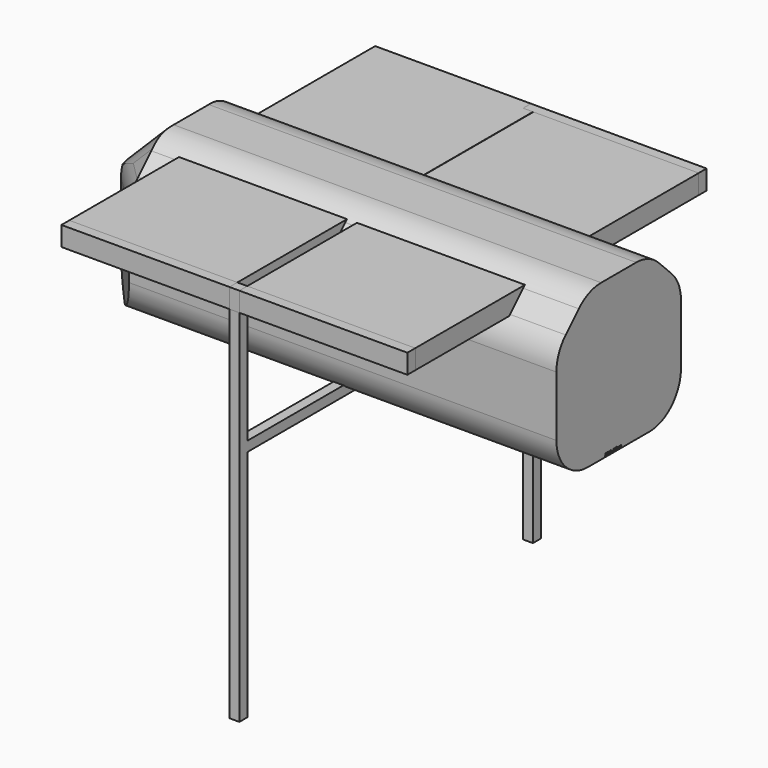
from build123d import *

# Parameters (mm, degrees)
F0_W          = 60
F0_H          = 20
F1_DEPTH      = 20
F3_DEPTH      = 15
F4_W          = 1.27
F4_H          = 1.2760577956
F5_DEPTH      = 15
F6_SIZE       = 5.08
F7_T1_DEPTH   = 65.4410244843
F7_T3_DEPTH   = 35.24
F7_T5_DEPTH   = 15.2572709248
F7_T7_DEPTH   = 15.2572709248
F7_T9_DEPTH   = 15.2572709248
F7_T14_DEPTH  = 37.62
F7_T19_DEPTH  = 37.62
F7_T24_DEPTH  = 50.32
F7_T31_DEPTH  = 50.32
F7_T37_DEPTH  = 50.32
F7_T43_DEPTH  = 54.13
F7_T49_DEPTH  = 54.13
F7_T55_DEPTH  = 54.13
F7_T62_DEPTH  = 41.43
F7_T67_DEPTH  = 41.43
F7_T72_DEPTH  = 49.0533849818
F7_T78_DEPTH  = 49.0533849818
F7_T84_DEPTH  = 49.0533849818
F7_T91_DEPTH  = 36.3533849818
F7_T96_DEPTH  = 36.3533849818
F7_T101_DEPTH = 55.4
F7_T107_DEPTH = 55.4
F7_T113_DEPTH = 55.4
F7_T120_DEPTH = 55.4
F7_T126_DEPTH = 55.4
F8_W          = 1.27
F8_H          = 1.2682774665
F9_DEPTH      = 15
F11_DEPTH     = 15
F12_W         = 21.5925588459
F12_H         = 1.2682774665
F13_DEPTH     = 2.5
F12_W_2       = 21.582525562
F14_DEPTH     = 2.5
F15_W         = 1.27
F15_H         = 1.2682774665
F16_DEPTH     = 2.5
F17_TEXT_SIZE = 0.4920971959
F18_DEPTH     = 0.0762
F20_W         = 0.5079289762
F20_H         = 6.7302512803
F21_DEPTH     = 0.3
F20_W_2       = 0.5036335206
F22_DEPTH     = 0.3
F20_W_3       = 0.5054401644
F23_DEPTH     = 0.3
F24_W         = 21.5925588459
F24_H         = 2.5
F25_DEPTH     = 25.4
F26_W         = 21.582525562
F26_H         = 2.5
F27_DEPTH     = 25.4
F29_DEPTH     = 2.5
F30_DEPTH     = 2.5
F31_W         = 1.2604115901
F31_H         = 2.5
F32_DEPTH     = 21.2852
F33_W         = 21.2420127096
F33_H         = 2.5
F34_DEPTH     = 25.4
F35_W         = 1.27
F35_H         = 1.2808652225
F36_DEPTH     = 30
F37_W         = 1.2666150182
F37_H         = 1.2703096864
F38_DEPTH     = 30


# Not quite as in the source:
# - a fillet or chamfer that OpenCascade refuses, or shapes differently, is made with other operations: its cross-section is extruded or revolved along the edge and cut away or added
# - two fillets or chamfers of one size are made in one step
# - Text() gives the source's letters only with a copy of the font that has no kerning and outlines rounded to 1/6400 em; it was checked with that copy


with BuildPart() as f1:
    # F0 (on Top) → F1 (new body)
    with BuildSketch(Plane.XY):
        with Locations((-42.5960034877, 2.3662830142)):
            Rectangle(F0_W, F0_H)
    extrude(amount=F1_DEPTH)

    # F2 (on face) → F3 (join)
    with BuildSketch(Plane(origin=(0, 12.3662830142, 0), x_dir=(-1, 0, 0), z_dir=(0, 1, 0))):
        Polygon((42.5873547792, 1.2760577956), (42.5960034877, 0), (43.862618506, 0), (43.862618506, 1.2760577956), align=None)
    extrude(amount=F3_DEPTH)

    # F4 (on face) → F5 (join)
    with BuildSketch(Plane.XZ.offset(7.6337169858)):
        with Locations((-41.9610034877, 0.6380288978)):
            Rectangle(F4_W, F4_H)
    extrude(amount=F5_DEPTH)

    # F6
    f6_edges = [f1.edges().sort_by_distance(p)[0] for p in [
        (-72.596003, 2.366283, 20),
        (-42.596003, -7.633717, 20),
        (-42.596003, 12.366283, 20),
        (-72.596003, 12.366283, 10),
        (-72.596003, -7.633717, 10),
    ]]
    chamfer(f6_edges, length=F6_SIZE)

    # F7: fillet of radius 5.08 on 13 edges, made by hand

    # F7_s2 → F7_t1 (cut)
    with BuildSketch(Plane.YZ.offset(-72.7765157298)):
        with BuildLine():
            ThreePointArc((5.1820781173, 20), (7.1261099537, 19.6133080252), (8.7741805657, 18.5121024484))
            Line((8.7741805657, 18.5121024484), (7.2862830142, 20))
            Line((7.2862830142, 20), (5.1820781173, 20))
        make_face()
        with BuildLine():
            ThreePointArc((12.3662830142, 12.8157951031), (11.9795910393, 14.7598269396), (10.8783854626, 16.4078975516))
            Line((10.8783854626, 16.4078975516), (12.3662830142, 14.92))
            Line((12.3662830142, 14.92), (12.3662830142, 12.8157951031))
        make_face()
        with BuildLine():
            ThreePointArc((-4.0416145374, 18.5121024484), (-2.3935439254, 19.6133080252), (-0.449512089, 20))
            Line((-0.449512089, 20), (-2.5537169858, 20))
            Line((-2.5537169858, 20), (-4.0416145374, 18.5121024484))
        make_face()
        with BuildLine():
            ThreePointArc((-7.6337169858, 12.8157951031), (-7.247025011, 14.7598269396), (-6.1458194343, 16.4078975516))
            Line((-6.1458194343, 16.4078975516), (-7.6337169858, 14.92))
            Line((-7.6337169858, 14.92), (-7.6337169858, 12.8157951031))
        make_face()
    extrude(amount=F7_T1_DEPTH, mode=Mode.SUBTRACT)

    # F7_s4 → F7_t3 (cut)
    with BuildSketch(Plane.XZ.offset(-19.9862830142)):
        with BuildLine():
            ThreePointArc((-67.5160034877, 0), (-71.1081059361, 1.4878975516), (-72.5960034877, 5.08))
            Line((-72.5960034877, 5.08), (-72.5960034877, 0))
            Line((-72.5960034877, 0), (-67.5160034877, 0))
        make_face()
    extrude(amount=F7_T3_DEPTH, mode=Mode.SUBTRACT)

    # F7_s6 → F7_t5 (cut)
    with BuildSketch(Plane(origin=(-27.0868833843, 27.0868833843, 0), x_dir=(0, 0, 1), z_dir=(-0.7071067812, 0.7071067812, 0))):
        with BuildLine():
            ThreePointArc((13.3053867944, -53.1388769511), (14.8441464628, -52.9002216696), (16.2383261619, -52.2066795822))
            Line((16.2383261619, -52.2066795822), (14.92, -53.1388769511))
            Line((14.92, -53.1388769511), (13.3053867944, -53.1388769511))
        make_face()
    extrude(amount=F7_T5_DEPTH, mode=Mode.SUBTRACT)

    # F7_s8 → F7_t7 (cut)
    with BuildSketch(Plane(origin=(-20.9037418772, 0, -20.9037418772), x_dir=(0, 1, 0), z_dir=(-0.7071067812, 0, -0.7071067812))):
        with BuildLine():
            ThreePointArc((-3.8720431477, -60.9509621596), (-2.4778634486, -61.644504247), (-0.9391037802, -61.8831595285))
            Line((-0.9391037802, -61.8831595285), (-2.5537169858, -61.8831595285))
            Line((-2.5537169858, -61.8831595285), (-3.8720431477, -60.9509621596))
        make_face()
        with BuildLine():
            ThreePointArc((5.6716698086, -61.8831595285), (7.2104294769, -61.644504247), (8.6046091761, -60.9509621596))
            Line((8.6046091761, -60.9509621596), (7.2862830142, -61.8831595285))
            Line((7.2862830142, -61.8831595285), (5.6716698086, -61.8831595285))
        make_face()
    extrude(amount=F7_T7_DEPTH, mode=Mode.SUBTRACT)

    # F7_s10 → F7_t9 (cut)
    with BuildSketch(Plane(origin=(-24.7206003701, -24.7206003701, 0), x_dir=(0, 0, 1), z_dir=(-0.7071067812, -0.7071067812, 0))):
        with BuildLine():
            ThreePointArc((13.3053867944, 56.4853064822), (14.8441464628, 56.2466512006), (16.2383261619, 55.5531091133))
            Line((16.2383261619, 55.5531091133), (14.92, 56.4853064822))
            Line((14.92, 56.4853064822), (13.3053867944, 56.4853064822))
        make_face()
    extrude(amount=F7_T9_DEPTH, mode=Mode.SUBTRACT)


with BuildPart() as f7_tool12:
    # F7_s13 → F7_t14 (new body)
    with BuildSketch(Plane.YZ.offset(-80.2160034877)):
        with BuildLine():
            ThreePointArc((-7.6337169858, 5.08), (-6.1458194343, 1.4878975516), (-2.5537169858, 0))
            Line((-2.5537169858, 0), (-7.6337169858, 0))
            Line((-7.6337169858, 0), (-7.6337169858, 5.08))
        make_face()
    extrude(amount=F7_T14_DEPTH)

    split(bisect_by=Plane.XY.offset(1.2760577956), keep=Keep.TOP)


with BuildPart() as f1_1:
    add(f1.part)

    # F7_t11: cut F7_tool12
    add(f7_tool12.part, mode=Mode.SUBTRACT)


with BuildPart() as f7_tool17:
    # F7_s18 → F7_t19 (new body)
    with BuildSketch(Plane.YZ.offset(-80.2160034877)):
        with BuildLine():
            ThreePointArc((-7.6337169858, 5.08), (-6.1458194343, 1.4878975516), (-2.5537169858, 0))
            Line((-2.5537169858, 0), (-7.6337169858, 0))
            Line((-7.6337169858, 0), (-7.6337169858, 5.08))
        make_face()
    extrude(amount=F7_T19_DEPTH)

    split(bisect_by=Plane.XY.offset(1.2760577956), keep=Keep.BOTTOM)


with BuildPart() as f1_2:
    add(f1_1.part)

    # F7_t16: cut F7_tool17
    add(f7_tool17.part, mode=Mode.SUBTRACT)


with BuildPart() as f7_tool22:
    # F7_s23 → F7_t24 (new body)
    with BuildSketch(Plane.YZ.offset(-80.2160034877)):
        with BuildLine():
            ThreePointArc((-7.6337169858, 5.08), (-6.1458194343, 1.4878975516), (-2.5537169858, 0))
            Line((-2.5537169858, 0), (-7.6337169858, 0))
            Line((-7.6337169858, 0), (-7.6337169858, 5.08))
        make_face()
    extrude(amount=F7_T24_DEPTH)

    split(bisect_by=Plane.YZ.offset(-42.5960034877), keep=Keep.TOP)

    split(bisect_by=Plane.XY.offset(1.2760577956), keep=Keep.TOP)

    split(bisect_by=Plane.YZ.offset(-41.3260034877), keep=Keep.BOTTOM)


with BuildPart() as f1_3:
    add(f1_2.part)

    # F7_t21: cut F7_tool22
    add(f7_tool22.part, mode=Mode.SUBTRACT)


with BuildPart() as f7_tool29:
    # F7_s30 → F7_t31 (new body)
    with BuildSketch(Plane.YZ.offset(-80.2160034877)):
        with BuildLine():
            ThreePointArc((-7.6337169858, 5.08), (-6.1458194343, 1.4878975516), (-2.5537169858, 0))
            Line((-2.5537169858, 0), (-7.6337169858, 0))
            Line((-7.6337169858, 0), (-7.6337169858, 5.08))
        make_face()
    extrude(amount=F7_T31_DEPTH)

    split(bisect_by=Plane.XY.offset(1.2760577956), keep=Keep.TOP)

    split(bisect_by=Plane.YZ.offset(-41.3260034877), keep=Keep.TOP)


with BuildPart() as f1_4:
    add(f1_3.part)

    # F7_t28: cut F7_tool29
    add(f7_tool29.part, mode=Mode.SUBTRACT)


with BuildPart() as f7_tool35:
    # F7_s36 → F7_t37 (new body)
    with BuildSketch(Plane.YZ.offset(-80.2160034877)):
        with BuildLine():
            ThreePointArc((-7.6337169858, 5.08), (-6.1458194343, 1.4878975516), (-2.5537169858, 0))
            Line((-2.5537169858, 0), (-7.6337169858, 0))
            Line((-7.6337169858, 0), (-7.6337169858, 5.08))
        make_face()
    extrude(amount=F7_T37_DEPTH)

    split(bisect_by=Plane.XY.offset(1.2760577956), keep=Keep.BOTTOM)

    split(bisect_by=Plane.YZ.offset(-41.3260034877), keep=Keep.TOP)


with BuildPart() as f1_5:
    add(f1_4.part)

    # F7_t34: cut F7_tool35
    add(f7_tool35.part, mode=Mode.SUBTRACT)


with BuildPart() as f7_tool41:
    # F7_s42 → F7_t43 (new body)
    with BuildSketch(Plane.YZ.offset(-54.0260034877)):
        with BuildLine():
            ThreePointArc((-7.6337169858, 5.08), (-6.1458194343, 1.4878975516), (-2.5537169858, 0))
            Line((-2.5537169858, 0), (-7.6337169858, 0))
            Line((-7.6337169858, 0), (-7.6337169858, 5.08))
        make_face()
    extrude(amount=F7_T43_DEPTH)

    split(bisect_by=Plane.YZ.offset(-42.5960034877), keep=Keep.BOTTOM)

    split(bisect_by=Plane.XY.offset(1.2760577956), keep=Keep.TOP)


with BuildPart() as f1_6:
    add(f1_5.part)

    # F7_t40: cut F7_tool41
    add(f7_tool41.part, mode=Mode.SUBTRACT)


with BuildPart() as f7_tool47:
    # F7_s48 → F7_t49 (new body)
    with BuildSketch(Plane.YZ.offset(-54.0260034877)):
        with BuildLine():
            ThreePointArc((-7.6337169858, 5.08), (-6.1458194343, 1.4878975516), (-2.5537169858, 0))
            Line((-2.5537169858, 0), (-7.6337169858, 0))
            Line((-7.6337169858, 0), (-7.6337169858, 5.08))
        make_face()
    extrude(amount=F7_T49_DEPTH)

    split(bisect_by=Plane.YZ.offset(-42.5960034877), keep=Keep.BOTTOM)

    split(bisect_by=Plane.XY.offset(1.2760577956), keep=Keep.BOTTOM)


with BuildPart() as f1_7:
    add(f1_6.part)

    # F7_t46: cut F7_tool47
    add(f7_tool47.part, mode=Mode.SUBTRACT)


with BuildPart() as f7_tool53:
    # F7_s54 → F7_t55 (new body)
    with BuildSketch(Plane.YZ.offset(-54.0260034877)):
        with BuildLine():
            ThreePointArc((-7.6337169858, 5.08), (-6.1458194343, 1.4878975516), (-2.5537169858, 0))
            Line((-2.5537169858, 0), (-7.6337169858, 0))
            Line((-7.6337169858, 0), (-7.6337169858, 5.08))
        make_face()
    extrude(amount=F7_T55_DEPTH)

    split(bisect_by=Plane.YZ.offset(-42.5960034877), keep=Keep.TOP)

    split(bisect_by=Plane.XY.offset(1.2760577956), keep=Keep.TOP)

    split(bisect_by=Plane.YZ.offset(-41.3260034877), keep=Keep.BOTTOM)


with BuildPart() as f1_8:
    add(f1_7.part)

    # F7_t52: cut F7_tool53
    add(f7_tool53.part, mode=Mode.SUBTRACT)


with BuildPart() as f7_tool60:
    # F7_s61 → F7_t62 (new body)
    with BuildSketch(Plane.YZ.offset(-41.3260034877)):
        with BuildLine():
            ThreePointArc((-7.6337169858, 5.08), (-6.1458194343, 1.4878975516), (-2.5537169858, 0))
            Line((-2.5537169858, 0), (-7.6337169858, 0))
            Line((-7.6337169858, 0), (-7.6337169858, 5.08))
        make_face()
    extrude(amount=F7_T62_DEPTH)

    split(bisect_by=Plane.XY.offset(1.2760577956), keep=Keep.TOP)


with BuildPart() as f1_9:
    add(f1_8.part)

    # F7_t59: cut F7_tool60
    add(f7_tool60.part, mode=Mode.SUBTRACT)


with BuildPart() as f7_tool65:
    # F7_s66 → F7_t67 (new body)
    with BuildSketch(Plane.YZ.offset(-41.3260034877)):
        with BuildLine():
            ThreePointArc((-7.6337169858, 5.08), (-6.1458194343, 1.4878975516), (-2.5537169858, 0))
            Line((-2.5537169858, 0), (-7.6337169858, 0))
            Line((-7.6337169858, 0), (-7.6337169858, 5.08))
        make_face()
    extrude(amount=F7_T67_DEPTH)

    split(bisect_by=Plane.XY.offset(1.2760577956), keep=Keep.BOTTOM)


with BuildPart() as f1_10:
    add(f1_9.part)

    # F7_t64: cut F7_tool65
    add(f7_tool65.part, mode=Mode.SUBTRACT)


with BuildPart() as f7_tool70:
    # F7_s71 → F7_t72 (new body)
    with BuildSketch(Plane.YZ.offset(-31.162618506)):
        with BuildLine():
            ThreePointArc((7.2862830142, 0), (10.8783854626, 1.4878975516), (12.3662830142, 5.08))
            Line((12.3662830142, 5.08), (12.3662830142, 0))
            Line((12.3662830142, 0), (7.2862830142, 0))
        make_face()
    extrude(amount=-F7_T72_DEPTH)

    split(bisect_by=Plane.XY.offset(1.2760577956), keep=Keep.BOTTOM)

    split(bisect_by=Plane(origin=(-42.5940468486, 0, 0.2886887214), x_dir=(0, 1, 0), z_dir=(0.9999770323, 0, -0.006777522)), keep=Keep.TOP)


with BuildPart() as f1_11:
    add(f1_10.part)

    # F7_t69: cut F7_tool70
    add(f7_tool70.part, mode=Mode.SUBTRACT)


with BuildPart() as f7_tool76:
    # F7_s77 → F7_t78 (new body)
    with BuildSketch(Plane.YZ.offset(-31.162618506)):
        with BuildLine():
            ThreePointArc((7.2862830142, 0), (10.8783854626, 1.4878975516), (12.3662830142, 5.08))
            Line((12.3662830142, 5.08), (12.3662830142, 0))
            Line((12.3662830142, 0), (7.2862830142, 0))
        make_face()
    extrude(amount=-F7_T78_DEPTH)

    split(bisect_by=Plane.XY.offset(1.2760577956), keep=Keep.TOP)

    split(bisect_by=Plane(origin=(-42.5940468486, 0, 0.2886887214), x_dir=(0, 1, 0), z_dir=(0.9999770323, 0, -0.006777522)), keep=Keep.TOP)


with BuildPart() as f1_12:
    add(f1_11.part)

    # F7_t75: cut F7_tool76
    add(f7_tool76.part, mode=Mode.SUBTRACT)


with BuildPart() as f7_tool82:
    # F7_s83 → F7_t84 (new body)
    with BuildSketch(Plane.YZ.offset(-31.162618506)):
        with BuildLine():
            ThreePointArc((7.2862830142, 0), (10.8783854626, 1.4878975516), (12.3662830142, 5.08))
            Line((12.3662830142, 5.08), (12.3662830142, 0))
            Line((12.3662830142, 0), (7.2862830142, 0))
        make_face()
    extrude(amount=-F7_T84_DEPTH)

    split(bisect_by=Plane.YZ.offset(-43.862618506), keep=Keep.TOP)

    split(bisect_by=Plane.XY.offset(1.2760577956), keep=Keep.TOP)

    split(bisect_by=Plane(origin=(-42.5940468486, 0, 0.2886887214), x_dir=(0, 1, 0), z_dir=(-0.9999770323, 0, 0.006777522)), keep=Keep.TOP)


with BuildPart() as f1_13:
    add(f1_12.part)

    # F7_t81: cut F7_tool82
    add(f7_tool82.part, mode=Mode.SUBTRACT)


with BuildPart() as f7_tool89:
    # F7_s90 → F7_t91 (new body)
    with BuildSketch(Plane.YZ.offset(-43.862618506)):
        with BuildLine():
            ThreePointArc((7.2862830142, 0), (10.8783854626, 1.4878975516), (12.3662830142, 5.08))
            Line((12.3662830142, 5.08), (12.3662830142, 0))
            Line((12.3662830142, 0), (7.2862830142, 0))
        make_face()
    extrude(amount=-F7_T91_DEPTH)

    split(bisect_by=Plane.XY.offset(1.2760577956), keep=Keep.BOTTOM)


with BuildPart() as f1_14:
    add(f1_13.part)

    # F7_t88: cut F7_tool89
    add(f7_tool89.part, mode=Mode.SUBTRACT)


with BuildPart() as f7_tool94:
    # F7_s95 → F7_t96 (new body)
    with BuildSketch(Plane.YZ.offset(-43.862618506)):
        with BuildLine():
            ThreePointArc((7.2862830142, 0), (10.8783854626, 1.4878975516), (12.3662830142, 5.08))
            Line((12.3662830142, 5.08), (12.3662830142, 0))
            Line((12.3662830142, 0), (7.2862830142, 0))
        make_face()
    extrude(amount=-F7_T96_DEPTH)

    split(bisect_by=Plane.XY.offset(1.2760577956), keep=Keep.TOP)


with BuildPart() as f1_15:
    add(f1_14.part)

    # F7_t93: cut F7_tool94
    add(f7_tool94.part, mode=Mode.SUBTRACT)


with BuildPart() as f7_tool99:
    # F7_s100 → F7_t101 (new body)
    with BuildSketch(Plane.YZ.offset(0.1039965123)):
        with BuildLine():
            ThreePointArc((7.2862830142, 0), (10.8783854626, 1.4878975516), (12.3662830142, 5.08))
            Line((12.3662830142, 5.08), (12.3662830142, 0))
            Line((12.3662830142, 0), (7.2862830142, 0))
        make_face()
    extrude(amount=-F7_T101_DEPTH)

    split(bisect_by=Plane.XY.offset(1.2760577956), keep=Keep.BOTTOM)

    split(bisect_by=Plane(origin=(-42.5940468486, 0, 0.2886887214), x_dir=(0, 1, 0), z_dir=(0.9999770323, 0, -0.006777522)), keep=Keep.TOP)


with BuildPart() as f1_16:
    add(f1_15.part)

    # F7_t98: cut F7_tool99
    add(f7_tool99.part, mode=Mode.SUBTRACT)


with BuildPart() as f7_tool105:
    # F7_s106 → F7_t107 (new body)
    with BuildSketch(Plane.YZ.offset(0.1039965123)):
        with BuildLine():
            ThreePointArc((7.2862830142, 0), (10.8783854626, 1.4878975516), (12.3662830142, 5.08))
            Line((12.3662830142, 5.08), (12.3662830142, 0))
            Line((12.3662830142, 0), (7.2862830142, 0))
        make_face()
    extrude(amount=-F7_T107_DEPTH)

    split(bisect_by=Plane.XY.offset(1.2760577956), keep=Keep.TOP)

    split(bisect_by=Plane(origin=(-42.5940468486, 0, 0.2886887214), x_dir=(0, 1, 0), z_dir=(0.9999770323, 0, -0.006777522)), keep=Keep.TOP)


with BuildPart() as f1_17:
    add(f1_16.part)

    # F7_t104: cut F7_tool105
    add(f7_tool105.part, mode=Mode.SUBTRACT)


with BuildPart() as f7_tool111:
    # F7_s112 → F7_t113 (new body)
    with BuildSketch(Plane.YZ.offset(0.1039965123)):
        with BuildLine():
            ThreePointArc((7.2862830142, 0), (10.8783854626, 1.4878975516), (12.3662830142, 5.08))
            Line((12.3662830142, 5.08), (12.3662830142, 0))
            Line((12.3662830142, 0), (7.2862830142, 0))
        make_face()
    extrude(amount=-F7_T113_DEPTH)

    split(bisect_by=Plane.YZ.offset(-43.862618506), keep=Keep.TOP)

    split(bisect_by=Plane.XY.offset(1.2760577956), keep=Keep.TOP)

    split(bisect_by=Plane(origin=(-42.5940468486, 0, 0.2886887214), x_dir=(0, 1, 0), z_dir=(-0.9999770323, 0, 0.006777522)), keep=Keep.TOP)


with BuildPart() as f1_18:
    add(f1_17.part)

    # F7_t110: cut F7_tool111
    add(f7_tool111.part, mode=Mode.SUBTRACT)


with BuildPart() as f7_tool118:
    # F7_s119 → F7_t120 (new body)
    with BuildSketch(Plane.YZ.offset(0.1039965123)):
        with BuildLine():
            ThreePointArc((7.2862830142, 0), (10.8783854626, 1.4878975516), (12.3662830142, 5.08))
            Line((12.3662830142, 5.08), (12.3662830142, 0))
            Line((12.3662830142, 0), (7.2862830142, 0))
        make_face()
    extrude(amount=-F7_T120_DEPTH)

    split(bisect_by=Plane.YZ.offset(-43.862618506), keep=Keep.BOTTOM)

    split(bisect_by=Plane.XY.offset(1.2760577956), keep=Keep.BOTTOM)


with BuildPart() as f1_19:
    add(f1_18.part)

    # F7_t117: cut F7_tool118
    add(f7_tool118.part, mode=Mode.SUBTRACT)


with BuildPart() as f7_tool124:
    # F7_s125 → F7_t126 (new body)
    with BuildSketch(Plane.YZ.offset(0.1039965123)):
        with BuildLine():
            ThreePointArc((7.2862830142, 0), (10.8783854626, 1.4878975516), (12.3662830142, 5.08))
            Line((12.3662830142, 5.08), (12.3662830142, 0))
            Line((12.3662830142, 0), (7.2862830142, 0))
        make_face()
    extrude(amount=-F7_T126_DEPTH)

    split(bisect_by=Plane.YZ.offset(-43.862618506), keep=Keep.BOTTOM)

    split(bisect_by=Plane.XY.offset(1.2760577956), keep=Keep.TOP)


with BuildPart() as f1_20:
    add(f1_19.part)

    # F7_t123: cut F7_tool124
    add(f7_tool124.part, mode=Mode.SUBTRACT)

    # F8 (on face) → F9 (join)
    with BuildSketch(Plane.XY.offset(1.2760577956)):
        with Locations((-41.9610034877, -21.9995782526)):
            Rectangle(F8_W, F8_H)
    extrude(amount=F9_DEPTH)

    # F10 (on face) → F11 (join)
    with BuildSketch(Plane.XY.offset(1.2760577956)):
        Polygon((-43.6347052455, 27.3662830142), (-43.862618506, 27.3662830142), (-43.862618506, 26.1058714241), (-42.5873547792, 26.1058714241), (-42.5873547792, 27.3662830142), align=None)
    extrude(amount=F11_DEPTH)

    # F17 (on face) → F18 (join)
    with BuildSketch(Plane.YZ.offset(-12.5960034877)):
        with Locations((0.1588490704, 0.0860145883)):
            Text('Allah Akbar', F17_TEXT_SIZE, font='Open Sans', text_align=(TextAlign.LEFT, TextAlign.BOTTOM))
    extrude(amount=F18_DEPTH)

    # F20 (on face) → F21 (join)
    with BuildSketch(Plane(origin=(-72.5960034877, 0, 0), x_dir=(0, -1, 0), z_dir=(-1, 0, 0))):
        with Locations((-5.4177053205, 9.9402611543)):
            Rectangle(F20_W, F20_H)
    extrude(amount=F21_DEPTH)

    # F20 (on face) → F22 (join)
    with BuildSketch(Plane(origin=(-72.5960034877, 0, 0), x_dir=(0, -1, 0), z_dir=(-1, 0, 0))):
        with Locations((-2.0122149144, 9.9402611543)):
            Rectangle(F20_W_2, F20_H)
    extrude(amount=F22_DEPTH)

    # F20 (on face) → F23 (join)
    with BuildSketch(Plane(origin=(-72.5960034877, 0, 0), x_dir=(0, -1, 0), z_dir=(-1, 0, 0))):
        with Locations((1.1918238625, 9.9402611543)):
            Rectangle(F20_W_3, F20_H)
    extrude(amount=F23_DEPTH)


with BuildPart() as f13:
    # F12 (on face) → F13 (new body)
    with BuildSketch(Plane.XY.offset(16.2760577956)):
        with Locations((-53.3922829106, -21.9995782526)):
            Rectangle(F12_W, F12_H)
    extrude(amount=F13_DEPTH)


with BuildPart() as f14:
    # F12 (on face) → F14 (new body)
    with BuildSketch(Plane.XY.offset(16.2760577956)):
        with Locations((-30.5347407067, -21.9995782526)):
            Rectangle(F12_W_2, F12_H)
    extrude(amount=F14_DEPTH)


with BuildPart() as f16:
    # F15 (on face) → F16 (new body)
    with BuildSketch(Plane.XY.offset(16.2760577956)):
        with Locations((-41.9610034877, -21.9995782526)):
            Rectangle(F15_W, F15_H)
    extrude(amount=F16_DEPTH)


with BuildPart() as f25:
    # F24 (on face) → F25 (new body)
    with BuildSketch(Plane(origin=(0, -21.3654395193, 0), x_dir=(-1, 0, 0), z_dir=(0, 1, 0))):
        with Locations((53.3922829106, 17.5260577956)):
            Rectangle(F24_W, F24_H)
    extrude(amount=F25_DEPTH)


with BuildPart() as f27:
    # F26 (on face) → F27 (new body)
    with BuildSketch(Plane(origin=(0, -21.3654395193, 0), x_dir=(-1, 0, 0), z_dir=(0, 1, 0))):
        with Locations((30.5347407067, 17.5260577956)):
            Rectangle(F26_W, F26_H)
    extrude(amount=F27_DEPTH)


with BuildPart() as f29:
    # F28 (on face) → F29 (new body)
    with BuildSketch(Plane.XY.offset(16.2760577956)):
        Polygon((-42.5873547792, 2.002238296), (-42.5873547792, 26.1058714241), (-43.862618506, 26.1058714241), (-43.862618506, 27.3662830142), (-63.8818889856, 27.3662830142), (-63.8818889856, 2.002238296), align=None)
    extrude(amount=F29_DEPTH)


with BuildPart() as f30:
    # F30 (new): a face of the model
    f30_faces = [f1_20.part.faces().sort_by_distance(p)[0] for p in [
        (-43.2249866426, 26.7360772191, 16.2760577956),
    ]]
    extrude(f30_faces, amount=F30_DEPTH)

    # F31 (on face) → F32 (join)
    with BuildSketch(Plane.YZ.offset(-42.5873547792)):
        with Locations((26.7360772191, 17.5260577956)):
            Rectangle(F31_W, F31_H)
    extrude(amount=F32_DEPTH)


with BuildPart() as f34:
    # F33 (on face) → F34 (new body)
    with BuildSketch(Plane.XZ.offset(-26.1058714241)):
        with Locations((-31.923161134, 17.5260577956)):
            Rectangle(F33_W, F33_H)
    extrude(amount=F34_DEPTH)


with BuildPart() as f1_21:
    add(f1_20.part)

    # F35 (on face) → F36 (join)
    with BuildSketch(Plane(origin=(0, 0, 0), x_dir=(1, 0, 0), z_dir=(0, 0, -1))):
        with Locations((-41.9610034877, 21.9932843746)):
            Rectangle(F35_W, F35_H)
    extrude(amount=F36_DEPTH)

    # F37 (on face) → F38 (join)
    with BuildSketch(Plane(origin=(0, 0, 0), x_dir=(1, 0, 0), z_dir=(0, 0, -1))):
        with Locations((-43.2293109968, -26.731128171)):
            Rectangle(F37_W, F37_H)
    extrude(amount=F38_DEPTH)


solid = Compound([f13.part, f14.part, f16.part, f25.part, f27.part, f29.part, f30.part, f34.part, f1_21.part])
